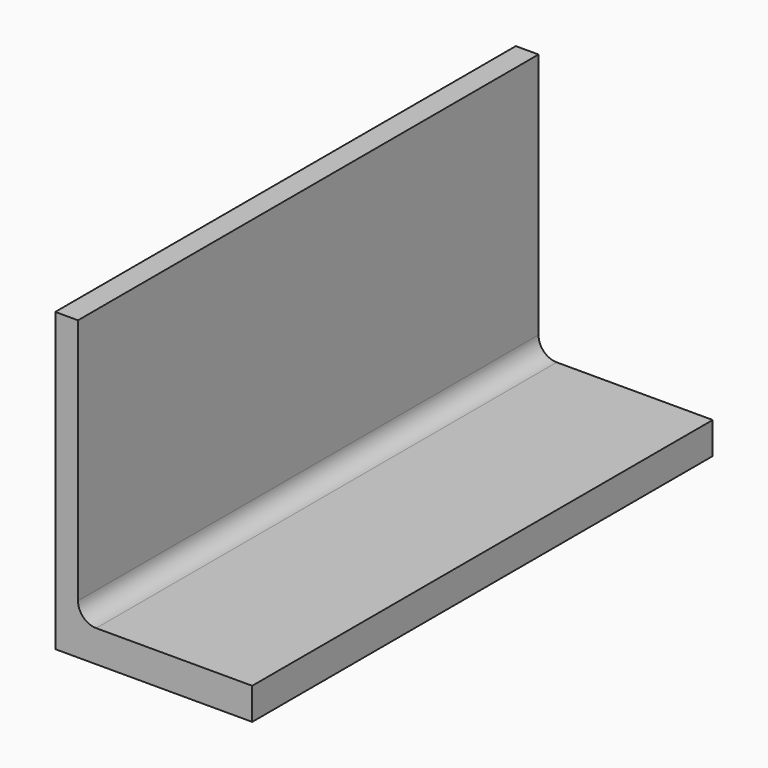
from build123d import *

# Parameters (mm, degrees)
F1_DEPTH = 190


# Not quite as in the source:
# - a feature names something its author has since deleted; it is built from what else it names


with BuildPart() as f1:
    # F0 (on Front) → F1 (new body)
    with BuildSketch(Plane.XZ):
        with BuildLine():
            Line((-32.5, -80), (32.5, -80))
            Line((32.5, -80), (32.5, -69.5))
            Line((32.5, -69.5), (-19, -69.5))
            ThreePointArc((-19, -69.5), (-23.2426406871, -67.7426406871), (-25, -63.5))
            Line((-25, -63.5), (-25, 18))
            Line((-25, 18), (-32.5, 18))
            Line((-32.5, 18), (-32.5, -80))
        make_face()
    extrude(amount=-F1_DEPTH)


solid = f1.part
